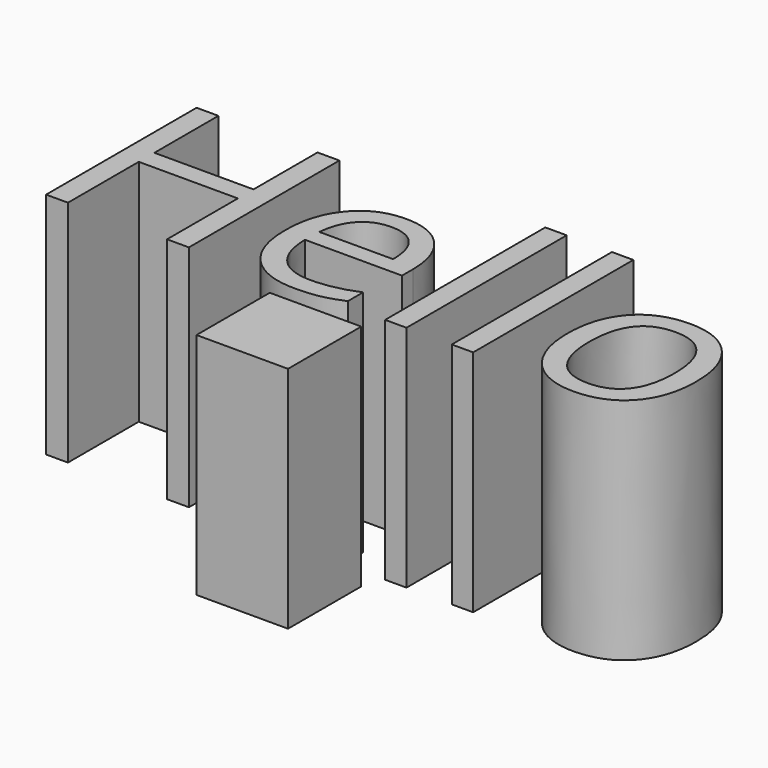
from build123d import *

# Parameters (mm, degrees)
F0_W         = 10
F0_H         = 10
F0_TEXT_SIZE = 28.7895297839
F1_DEPTH     = 25


# Not quite as in the source:
# - Text() gives the source's letters only with a copy of the font that has no kerning and outlines rounded to 1/6400 em; it was checked with that copy


with BuildPart() as f1:
    # F0 (on Top) → F1 (new body)
    with BuildSketch(Plane.XY):
        with Locations((5, 5)):
            Rectangle(F0_W, F0_H)
        with Locations((-29.0520247072, 12.2411809862)):
            Text('Hello', F0_TEXT_SIZE, font='Open Sans', text_align=(TextAlign.LEFT, TextAlign.BOTTOM))
    extrude(amount=F1_DEPTH)


solid = f1.part
